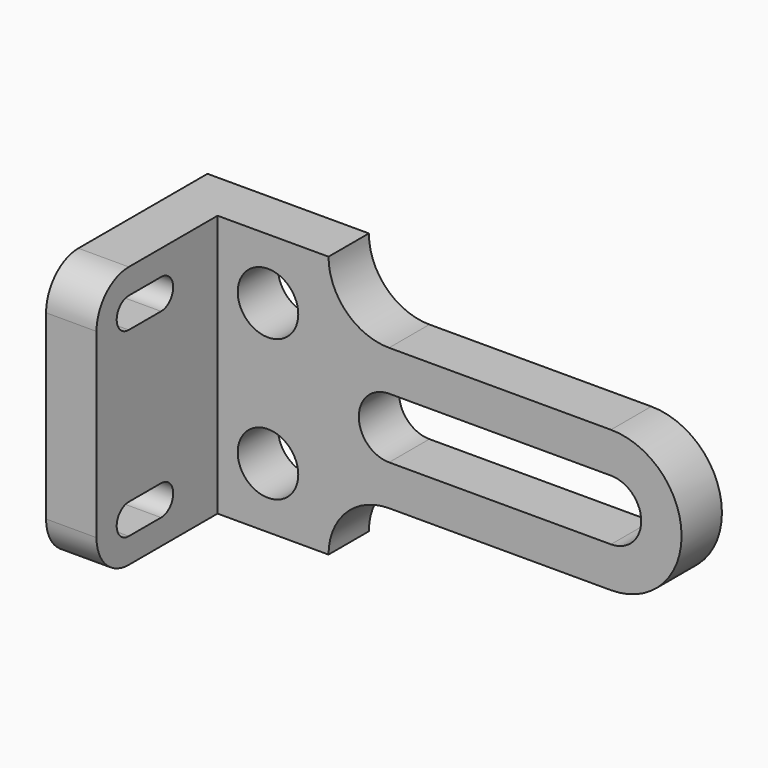
from build123d import *

# Parameters (mm, degrees)
F0_R     = 6
F1_DEPTH = 10
F2_W     = 40
F2_H     = 52
F3_DEPTH = 10
F4_R     = 11.99999
F5_R     = 8
F7_DEPTH = 102.001


# Not quite as in the source:
# - a fillet or chamfer is up to 0.001 mm smaller than in the source, because OpenCascade refuses the exact size


with BuildPart() as f1:
    # F0 (on Front) → F1 (new body)
    with BuildSketch(Plane.XZ):
        with BuildLine():
            Line((32, 52), (0, 52))
            Line((0, 52), (0, 0))
            Line((0, 0), (32, 0))
            Line((32, 0), (32, 12))
            Line((32, 12), (88, 12))
            ThreePointArc((88, 12), (102, 26), (88, 40))
            Line((88, 40), (32, 40))
            Line((32, 40), (32, 52))
        make_face()
        with Locations((20, 12)):
            Circle(F0_R, mode=Mode.SUBTRACT)
        with Locations((20, 40)):
            Circle(F0_R, mode=Mode.SUBTRACT)
        with BuildLine():
            ThreePointArc((44, 20), (38, 26), (44, 32))
            Line((44, 32), (88, 32))
            ThreePointArc((88, 32), (94, 26), (88, 20))
            Line((88, 20), (44, 20))
        make_face(mode=Mode.SUBTRACT)
    extrude(amount=F1_DEPTH)

    # F2 (on Right) → F3 (join)
    with BuildSketch(Plane.YZ):
        with Locations((-20, 26)):
            Rectangle(F2_W, F2_H)
    extrude(amount=F3_DEPTH)

    # F4 (radius 12 in the source; OpenCascade refuses exactly that, so slightly less here)
    f4_edges = [f1.edges().sort_by_distance(p)[0] for p in [
        (32, -5, 40),
        (32, -5, 12),
    ]]
    fillet(f4_edges, radius=F4_R)

    # F5
    f5_edges = [f1.edges().sort_by_distance(p)[0] for p in [
        (5, -40, 0),
        (5, -40, 52),
    ]]
    fillet(f5_edges, radius=F5_R)

    # F6 (on Right) → F7 (cut, through all)
    with BuildSketch(Plane.YZ):
        with BuildLine():
            Line((-24, 11), (-32, 11))
            ThreePointArc((-32, 11), (-35, 8), (-32, 5))
            Line((-32, 5), (-24, 5))
            ThreePointArc((-24, 5), (-21, 8), (-24, 11))
        make_face()
    extrude(amount=F7_DEPTH, mode=Mode.SUBTRACT)

    # F9: F1 across plane


with BuildPart() as f1_1:
    add(f1.part)
    add(f1.part.mirror(Plane(origin=(11.5185185185, -11.5185185185, 26), x_dir=(1, 0, 0), z_dir=(0, 0, 1))), mode=Mode.INTERSECT)


solid = f1_1.part
